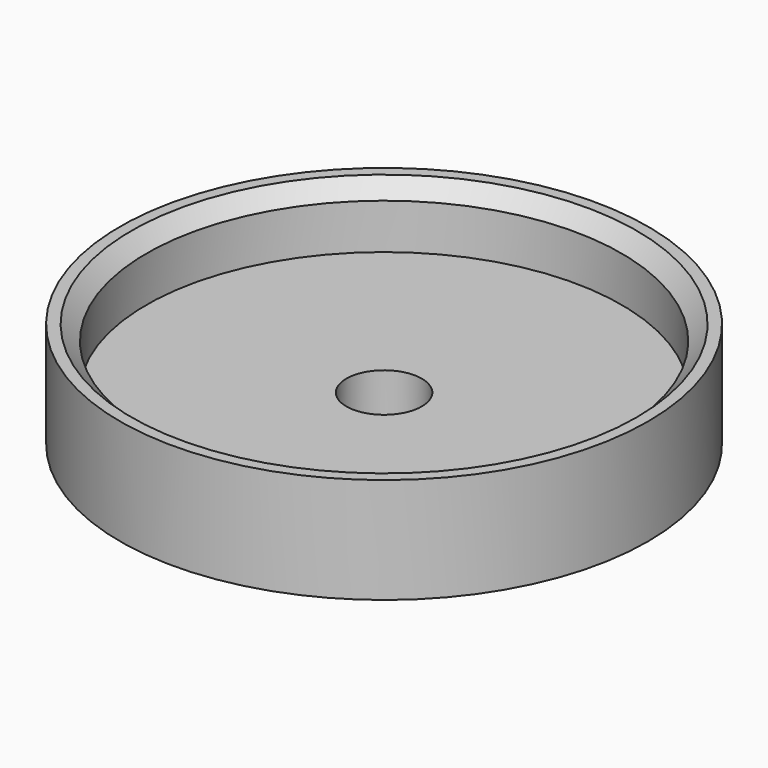
from build123d import *

# Parameters (mm, degrees)
F0_R     = 17.5
F0_R_2   = 15.75
F1_DEPTH = 7
F0_R_3   = 2.5
F2_DEPTH = 3
F3_SIZE  = 1


# Not quite as in the source:
# - a feature names something its author has since deleted; it is built from what else it names


with BuildPart() as f1:
    # F0 (on Top) → F1 (new body)
    with BuildSketch(Plane.XY):
        Circle(F0_R)
        Circle(F0_R_2, mode=Mode.SUBTRACT)
    extrude(amount=F1_DEPTH)

    # F0 (on Top) → F2 (join)
    with BuildSketch(Plane.XY):
        Circle(F0_R_2)
        Circle(F0_R_3, mode=Mode.SUBTRACT)
    extrude(amount=F2_DEPTH)

    # F3
    f3_edges = [f1.edges().sort_by_distance(p)[0] for p in [
        (-15.75, 0, 7),
    ]]
    chamfer(f3_edges, length=F3_SIZE)


solid = f1.part
